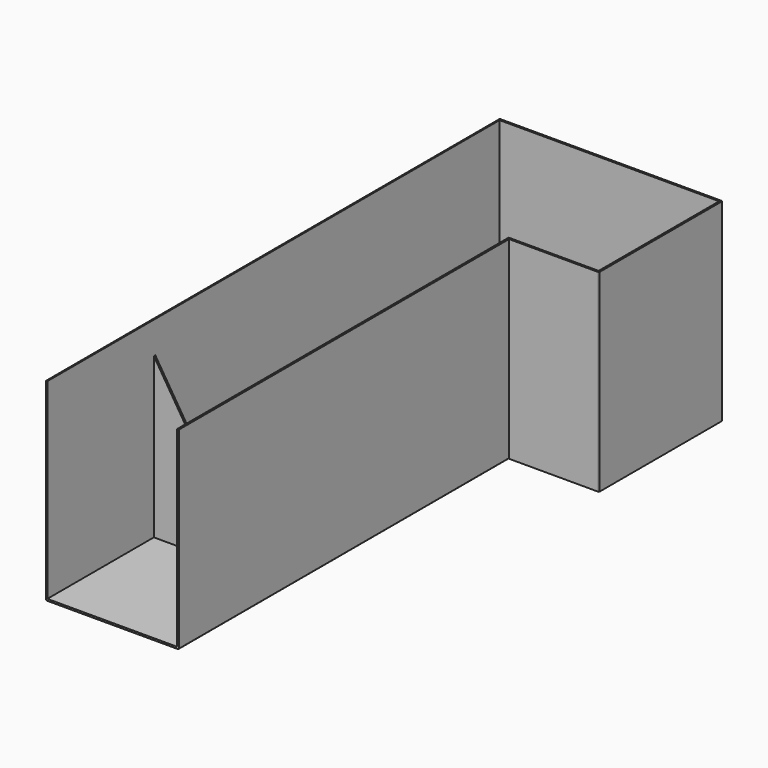
from build123d import *

# Parameters (mm, degrees)
F1_DEPTH  = 426
F3_DEPTH  = 4
F4_R      = 2
F7_DEPTH  = 4
F10_DEPTH = 4


# Not quite as in the source:
# - a feature names something its author has since deleted; it is built from what else it names


with BuildPart() as f1:
    # F0 (on Top) → F1 (new body)
    with BuildSketch(Plane.XY):
        Polygon((-200, -343), (0, -343), (0, 0), (-495, 0), (-495, -1261), (-492.1838745495, -1261), (-492.1838745495, -4), (-4, -4), (-4, -339), (-204, -339), (-204, -1261), (-200, -1261), align=None)
    extrude(amount=F1_DEPTH)

    # F2 (on Top) → F3 (join)
    with BuildSketch(Plane.XY):
        Polygon((0, 0), (-495, 0), (-495, -1261), (-200, -1261), (-200, -343), (0, -343), align=None)
    extrude(amount=-F3_DEPTH)

    # F4
    f4_edges = [f1.edges().sort_by_distance(p)[0] for p in [
        (-200, -802, -4),
        (-495, -630.5, -4),
        (-247.5, 0, -4),
        (0, -343, 211),
        (0, 0, 211),
    ]]
    fillet(f4_edges, radius=F4_R)

    # F6 (on offset) → F7 (join)
    with BuildSketch(Plane.XZ.offset(961)):
        Polygon((-492.1838745495, 355), (-492.1838745495, 0), (-270.1838745495, 0), align=None)
    extrude(amount=F7_DEPTH)

    # F9 (on offset) → F10 (join)
    with BuildSketch(Plane.XZ.offset(361)):
        Polygon((-204, 355), (-426, 0), (-204, 0), align=None)
    extrude(amount=F10_DEPTH)


solid = f1.part
